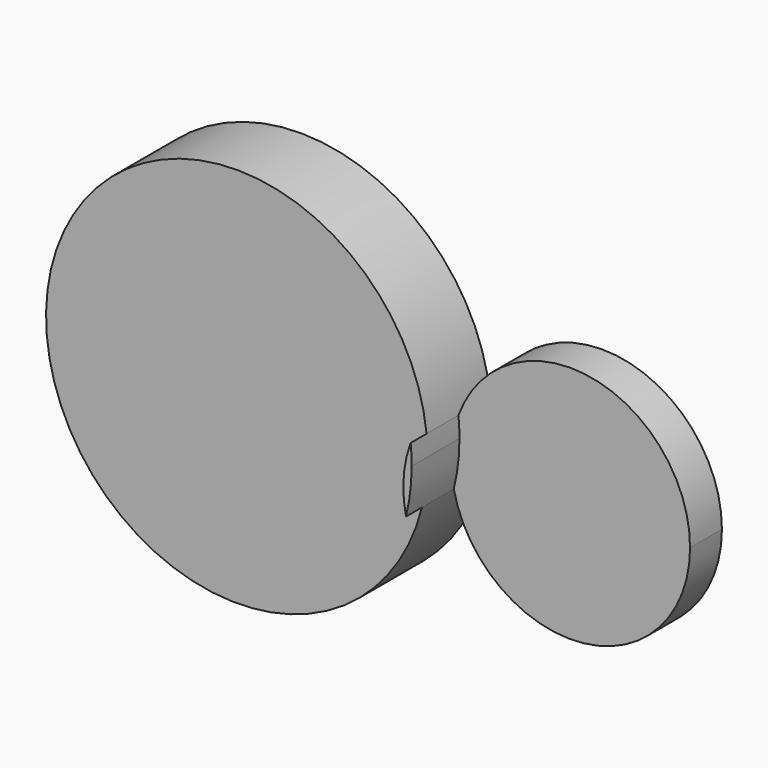
from build123d import *
from build123d import SkipClean  # not in build123d's __all__

# Parameters (mm, degrees)
F1_DEPTH = 25.4
F2_DEPTH = 31.75
F3_DEPTH = 12.7


with BuildPart() as f1:
    # F0 (on Front) → F1 (new body)
    with BuildSketch(Plane.XZ):
        with BuildLine():
            ThreePointArc((-37.244253, -8.029669), (-38.007654, 2.651088), (-35.768864, 13.122439))
            ThreePointArc((-35.768864, 13.122439), (-156.95564, 10.947881), (-37.244253, -8.029669))
        make_face()
    extrude(amount=F1_DEPTH)

    # F0 (on Front) → F2 (join, symmetric)
    with BuildSketch(Plane.XZ):
        with BuildLine():
            ThreePointArc((-35.430472, 6.714746), (-35.515129, 9.923057), (-35.768864, 13.122439))
            ThreePointArc((-35.768864, 13.122439), (-38.007654, 2.651088), (-37.244253, -8.029669))
            ThreePointArc((-37.244253, -8.029669), (-35.88562, -0.713032), (-35.430472, 6.714746))
        make_face()
    extrude(amount=F2_DEPTH, both=True)

    # F0 (on Front) → F3 (join)
    with BuildSketch(Plane.XZ):
        with BuildLine():
            ThreePointArc((-37.244253, -8.029669), (4.03757, -37.885459), (38.1, 0))
            ThreePointArc((38.1, 0), (6.663944, 37.512689), (-35.768864, 13.122439))
            ThreePointArc((-35.768864, 13.122439), (-35.515129, 9.923057), (-35.430472, 6.714746))
            ThreePointArc((-35.430472, 6.714746), (-35.88562, -0.713032), (-37.244253, -8.029669))
        make_face()
    with SkipClean():  # cleaning this boolean's faces spoils the solid; the shape is the same uncleaned
        extrude(amount=F3_DEPTH)


solid = f1.part
